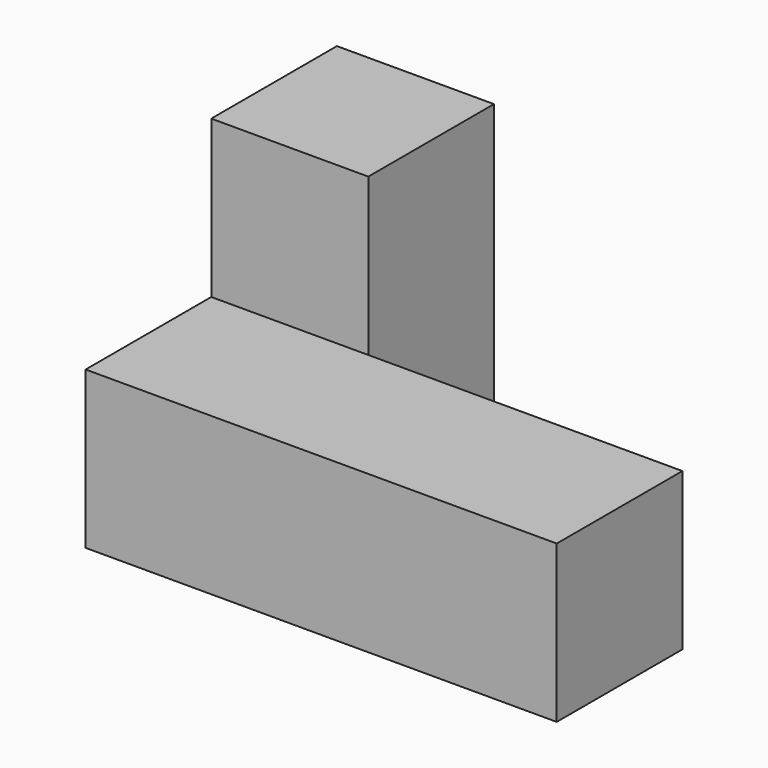
from build123d import *

# Parameters (mm, degrees)
F1_W     = 228.6
F1_H     = 76.2
F2_DEPTH = 76.2
F3_W     = 76.2
F3_H     = 76.2
F4_DEPTH = 76.2
F5_W     = 76.2
F5_H     = 76.2
F6_DEPTH = 76.2


# Not quite as in the source:
# - a variable given as a bare number and used for a length is read in inches; the dataset says mm whatever the document's units were


with BuildPart() as f2:
    # F1 (on Front) → F2 (new body)
    with BuildSketch(Plane.XZ):
        Rectangle(F1_W, F1_H)
    extrude(amount=F2_DEPTH)

    # F3 (on face) → F4 (join)
    with BuildSketch(Plane(origin=(0, 0, 0), x_dir=(-1, 0, 0), z_dir=(0, 1, 0))):
        with Locations((76.2, 0)):
            Rectangle(F3_W, F3_H)
    extrude(amount=F4_DEPTH)

    # F5 (on face) → F6 (join)
    with BuildSketch(Plane.XY.offset(38.1)):
        with Locations((-76.2, 38.1)):
            Rectangle(F5_W, F5_H)
    extrude(amount=F6_DEPTH)


solid = f2.part
